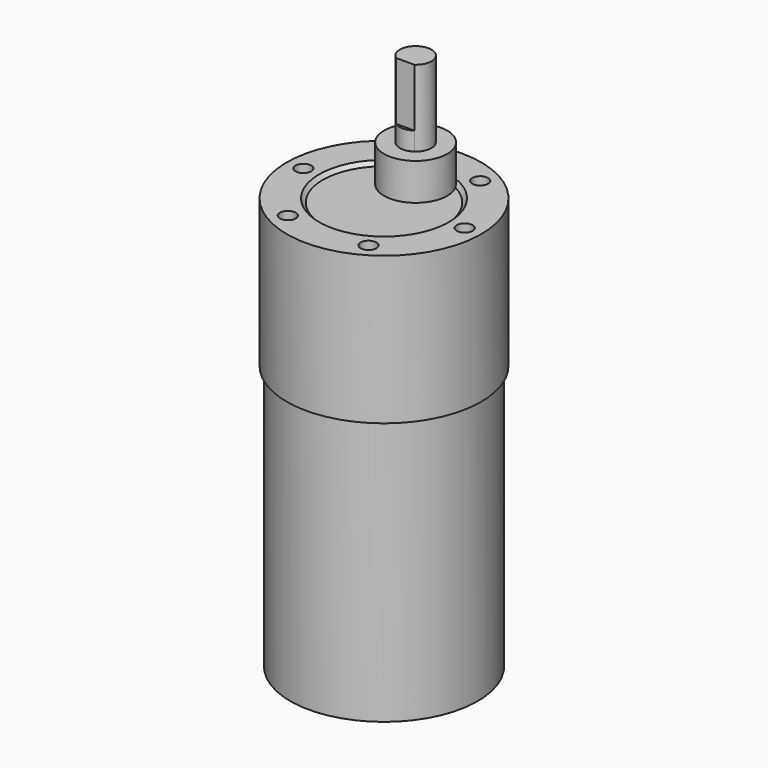
from build123d import *

# Parameters (mm, degrees)
F2_R      = 6
F3_DEPTH  = 7
F4_SIZE   = 0.69999
F5_R      = 1.5
F6_DEPTH  = 5
F8_DEPTH  = 14.5
F9_R      = 3
F10_DEPTH = 3.5


# Not quite as in the source:
# - a fillet or chamfer is up to 0.001 mm smaller than in the source, because OpenCascade refuses the exact size


with BuildPart() as f1:
    # F0 (on Right) → F1 (revolve)
    with BuildSketch(Plane.YZ):
        Polygon((0, 77.5), (0, 0), (17.8, 0), (17.8, 50.2), (18.45, 50.2), (18.45, 78.2), (12.3, 78.2), (12.3, 77.5), align=None)
    revolve(axis=Axis((0, 0, 6.0807448852), (0, 0, -1)))

    # F2 (on face) → F3 (join)
    with BuildSketch(Plane.XY.offset(77.5)):
        with Locations((0, 7.5)):
            Circle(F2_R)
    extrude(amount=F3_DEPTH)

    # F4 (size 0.7 in the source; OpenCascade refuses exactly that, so slightly less here)
    f4_edges = [f1.edges().sort_by_distance(p)[0] for p in [
        (0, -12.3, 77.5),
    ]]
    chamfer(f4_edges, length=F4_SIZE)

    # F5 (on face) → F6 (cut)
    with BuildSketch(Plane.XY.offset(78.2)):
        with Locations((-15.3, 0)):
            Circle(F5_R)
        with Locations((-7.65, -13.2501886779)):
            Circle(F5_R)
        with Locations((7.65, -13.2501886779)):
            Circle(F5_R)
        with Locations((15.3, 0)):
            Circle(F5_R)
        with Locations((7.65, 13.2501886779)):
            Circle(F5_R)
        with Locations((-7.65, 13.2501886779)):
            Circle(F5_R)
    extrude(amount=-F6_DEPTH, mode=Mode.SUBTRACT)


with BuildPart() as f8:
    # F7 (on face) → F8 (new body)
    with BuildSketch(Plane.XY.offset(84.5)):
        with BuildLine():
            Line((-1.7313289693, 5.05), (1.7313289693, 5.05))
            ThreePointArc((1.7313289693, 5.05), (0, 10.5), (-1.7313289693, 5.05))
        make_face()
    extrude(amount=F8_DEPTH)

    # F9 (on face) → F10 (join)
    with BuildSketch(Plane.XY.offset(84.5)):
        with Locations((0, 7.5)):
            Circle(F9_R)
    extrude(amount=F10_DEPTH)


solid = Compound([f1.part, f8.part])
